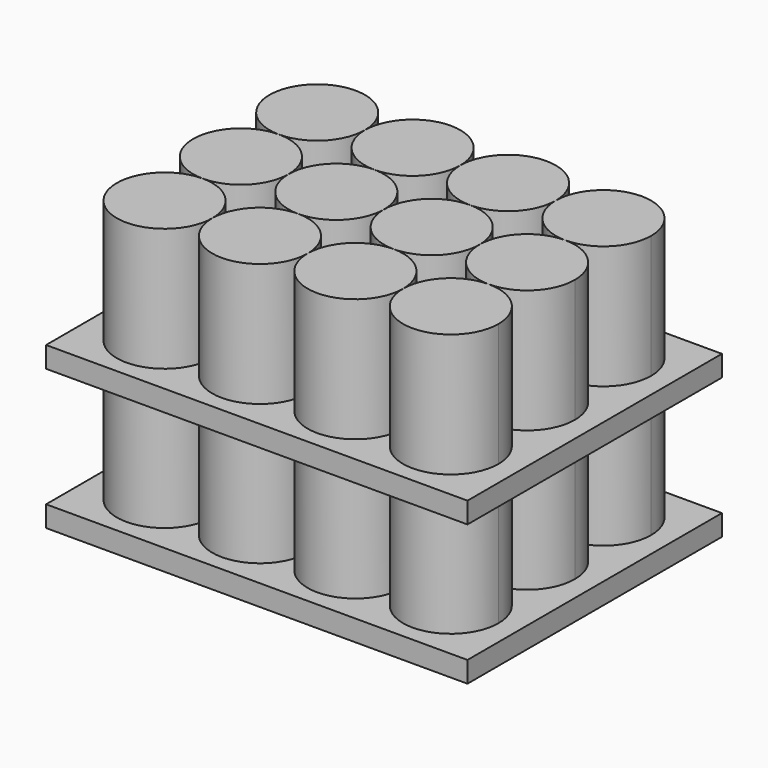
from build123d import *

# Parameters (mm, degrees)
F1_DEPTH = 84.1627984
F2_W     = 134.62
F2_H     = 6.6927933697
F3_DEPTH = 50.8
F2_H_2   = 6.6927984


# Not quite as in the source:
# - a feature names something its author has since deleted; it is built from what else it names


with BuildPart() as f1:
    # F0 (on Top) → F1 (new body)
    with BuildSketch(Plane.XY):
        with BuildLine():
            ThreePointArc((-45.72, -15.24), (-56.4963073453, -41.2563073453), (-30.48, -30.48))
            ThreePointArc((-30.48, -30.48), (-34.9436926547, -19.7036926547), (-45.72, -15.24))
        make_face()
    extrude(amount=F1_DEPTH)


with BuildPart() as f1b:
    # F0 (on Top) → F1, piece 2 (new body)
    with BuildSketch(Plane.XY):
        with BuildLine():
            ThreePointArc((-15.2399999801, -15.24), (-26.0163073382, -19.7036926477), (-30.48, -30.48))
            ThreePointArc((-30.48, -30.48), (-15.24, -45.72), (0, -30.48))
            ThreePointArc((0, -30.48), (-4.4636926477, -19.7036926618), (-15.2399999801, -15.24))
        make_face()
    extrude(amount=F1_DEPTH)


with BuildPart() as f1c:
    # F0 (on Top) → F1, piece 3 (new body)
    with BuildSketch(Plane.XY):
        with BuildLine():
            ThreePointArc((-45.72, 15.24), (-60.96, 0), (-45.72, -15.24))
            ThreePointArc((-45.72, -15.24), (-34.9436926547, -10.7763073453), (-30.48, 0))
            ThreePointArc((-30.48, 0), (-34.9436926547, 10.7763073453), (-45.72, 15.24))
        make_face()
    extrude(amount=F1_DEPTH)


with BuildPart() as f1d:
    # F0 (on Top) → F1, piece 4 (new body)
    with BuildSketch(Plane.XY):
        with BuildLine():
            ThreePointArc((15.2400000199, -15.24), (4.4636926618, -19.7036926477), (0, -30.48))
            ThreePointArc((0, -30.48), (15.24, -45.72), (30.48, -30.48))
            ThreePointArc((30.48, -30.48), (26.0163073523, -19.7036926618), (15.2400000199, -15.24))
        make_face()
    extrude(amount=F1_DEPTH)


with BuildPart() as f1e:
    # F0 (on Top) → F1, piece 5 (new body)
    with BuildSketch(Plane.XY):
        with BuildLine():
            ThreePointArc((-30.48, 0), (-26.0163073382, -10.7763073523), (-15.2399999801, -15.24))
            ThreePointArc((-15.2399999801, -15.24), (-4.4636926477, -10.7763073382), (0, 0))
            ThreePointArc((0, 0), (-4.4636926477, 10.7763073382), (-15.2399999801, 15.24))
            ThreePointArc((-15.2399999801, 15.24), (-26.0163073382, 10.7763073523), (-30.48, 0))
        make_face()
    extrude(amount=F1_DEPTH)


with BuildPart() as f1f:
    # F0 (on Top) → F1, piece 6 (new body)
    with BuildSketch(Plane.XY):
        with BuildLine():
            ThreePointArc((-30.48, 30.48), (-56.4963073453, 41.2563073453), (-45.72, 15.24))
            ThreePointArc((-45.72, 15.24), (-34.9436926547, 19.7036926547), (-30.48, 30.48))
        make_face()
    extrude(amount=F1_DEPTH)


with BuildPart() as f1g:
    # F0 (on Top) → F1, piece 7 (new body)
    with BuildSketch(Plane.XY):
        with BuildLine():
            ThreePointArc((45.7200000919, -15.24), (34.9436926872, -19.7036926222), (30.48, -30.48))
            ThreePointArc((30.48, -30.48), (45.72, -45.72), (60.96, -30.48))
            ThreePointArc((60.96, -30.48), (56.4963073778, -19.7036926872), (45.7200000919, -15.24))
        make_face()
    extrude(amount=F1_DEPTH)


with BuildPart() as f1h:
    # F0 (on Top) → F1, piece 8 (new body)
    with BuildSketch(Plane.XY):
        with BuildLine():
            ThreePointArc((0, 0), (4.4636926618, -10.7763073523), (15.2400000199, -15.24))
            ThreePointArc((15.2400000199, -15.24), (26.0163073523, -10.7763073382), (30.48, 0))
            ThreePointArc((30.48, 0), (26.0163073523, 10.7763073382), (15.2400000199, 15.24))
            ThreePointArc((15.2400000199, 15.24), (4.4636926618, 10.7763073523), (0, 0))
        make_face()
    extrude(amount=F1_DEPTH)


with BuildPart() as f1i:
    # F0 (on Top) → F1, piece 9 (new body)
    with BuildSketch(Plane.XY):
        with BuildLine():
            ThreePointArc((0, 30.48), (-15.24, 45.72), (-30.48, 30.48))
            ThreePointArc((-30.48, 30.48), (-26.0163073382, 19.7036926477), (-15.2399999801, 15.24))
            ThreePointArc((-15.2399999801, 15.24), (-4.4636926477, 19.7036926618), (0, 30.48))
        make_face()
    extrude(amount=F1_DEPTH)


with BuildPart() as f1j:
    # F0 (on Top) → F1, piece 10 (new body)
    with BuildSketch(Plane.XY):
        with BuildLine():
            ThreePointArc((30.48, 0), (34.9436926872, -10.7763073778), (45.7200000919, -15.24))
            ThreePointArc((45.7200000919, -15.24), (56.4963073778, -10.7763073128), (60.96, 0))
            ThreePointArc((60.96, 0), (56.4963073778, 10.7763073128), (45.7200000919, 15.24))
            ThreePointArc((45.7200000919, 15.24), (34.9436926872, 10.7763073778), (30.48, 0))
        make_face()
    extrude(amount=F1_DEPTH)


with BuildPart() as f1k:
    # F0 (on Top) → F1, piece 11 (new body)
    with BuildSketch(Plane.XY):
        with BuildLine():
            ThreePointArc((0, 30.48), (4.4636926618, 19.7036926477), (15.2400000199, 15.24))
            ThreePointArc((15.2400000199, 15.24), (26.0163073523, 19.7036926618), (30.48, 30.48))
            ThreePointArc((30.48, 30.48), (15.24, 45.72), (0, 30.48))
        make_face()
    extrude(amount=F1_DEPTH)


with BuildPart() as f1l:
    # F0 (on Top) → F1, piece 12 (new body)
    with BuildSketch(Plane.XY):
        with BuildLine():
            ThreePointArc((30.48, 30.48), (34.9436926872, 19.7036926222), (45.7200000919, 15.24))
            ThreePointArc((45.7200000919, 15.24), (56.4963073778, 19.7036926872), (60.96, 30.48))
            ThreePointArc((60.96, 30.48), (45.72, 45.72), (30.48, 30.48))
        make_face()
    extrude(amount=F1_DEPTH)


with BuildPart() as f3:
    # F2 (on Front) → F3 (new body, symmetric)
    with BuildSketch(Plane.XZ):
        with Locations((0, -3.3463966849)):
            Rectangle(F2_W, F2_H)
    extrude(amount=F3_DEPTH, both=True)


with BuildPart() as f3b:
    # F2 (on Front) → F3, piece 2 (new body, symmetric)
    with BuildSketch(Plane.XZ):
        with Locations((0, 41.4463992)):
            Rectangle(F2_W, F2_H_2)
    extrude(amount=F3_DEPTH, both=True)


solid = Compound([f1.part, f1b.part, f1c.part, f1d.part, f1e.part, f1f.part, f1g.part, f1h.part, f1i.part, f1j.part, f1k.part, f1l.part, f3.part, f3b.part])
